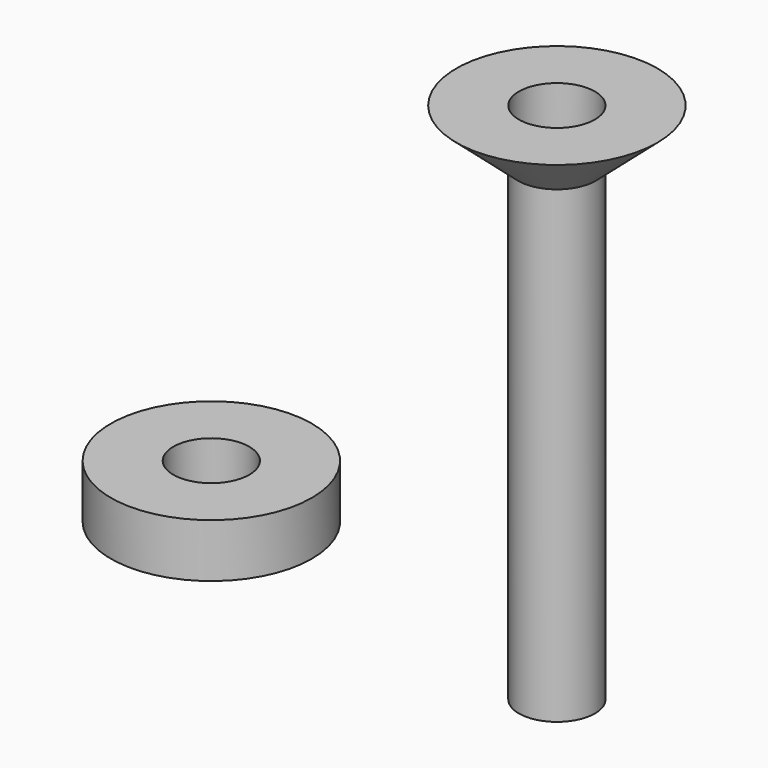
from build123d import *

# Parameters (mm, degrees)
F0_R      = 3.6000055
F1_DEPTH  = 44.45
F2_W      = 3.1999936
F2_H      = 3.1999936
F3_DEPTH  = 45.466
F4_R      = 9.525
F4_R_2    = 3.6000055
F5_DEPTH  = 5.08
F6_SIZE2  = 5.84199
F6_SIZE   = 5.07999
F7_R      = 9.525
F8_DEPTH  = 5.08
F9_R      = 3.60045
F10_DEPTH = 6.096


# Not quite as in the source:
# - a fillet or chamfer is up to 0.001 mm smaller than in the source, because OpenCascade refuses the exact size


with BuildPart() as f1:
    # F0 (on Top) → F1 (new body)
    with BuildSketch(Plane.XY):
        Circle(F0_R)
    extrude(amount=F1_DEPTH)

    # F2 (on face) → F3 (cut)
    with BuildSketch(Plane(origin=(0, 0, 0), x_dir=(1, 0, 0), z_dir=(0, 0, -1))):
        Rectangle(F2_W, F2_H)
    extrude(amount=-F3_DEPTH, mode=Mode.SUBTRACT)


with BuildPart() as f5:
    # F4 (on face) → F5 (new body)
    with BuildSketch(Plane.XY.offset(44.45)):
        Circle(F4_R)
        Circle(F4_R_2, mode=Mode.SUBTRACT)
    extrude(amount=F5_DEPTH)

    # F6 (size 5.08 and 5.842 in the source; OpenCascade refuses exactly that, so slightly less here)
    f6_edges = [f5.edges().sort_by_distance(p)[0] for p in [
        (-9.525, 0, 44.45),
    ]]
    f6_side = f5.faces().sort_by_distance((-9.525, 0, 46.99))[0]
    chamfer(f6_edges, length=F6_SIZE, length2=F6_SIZE2, reference=f6_side)


with BuildPart() as f8:
    # F7 (on Top) → F8 (new body)
    with BuildSketch(Plane.XY):
        with Locations((-37.7559922636, 6.275920663)):
            Circle(F7_R)
    extrude(amount=F8_DEPTH)

    # F9 (on face) → F10 (cut)
    with BuildSketch(Plane(origin=(0, 0, 0), x_dir=(1, 0, 0), z_dir=(0, 0, -1))):
        with Locations((-37.7559922636, -6.275920663)):
            Circle(F9_R)
    extrude(amount=-F10_DEPTH, mode=Mode.SUBTRACT)


solid = Compound([f1.part, f5.part, f8.part])
